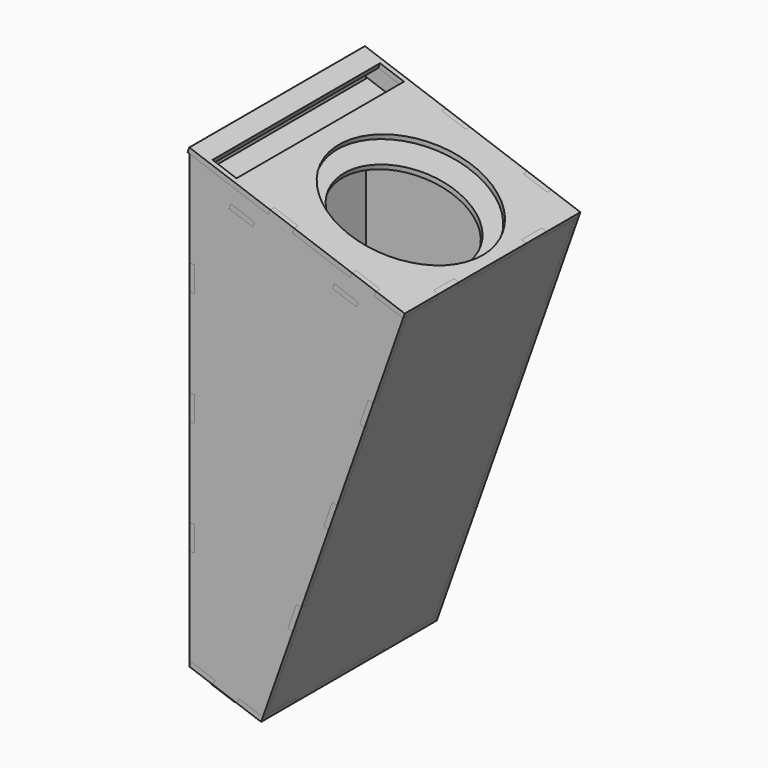
from build123d import *

# Parameters (mm, degrees)
F15_DEPTH = 2
F8_W      = 2
F8_H      = 10
F8_W_2    = 10
F8_H_2    = 2
F16_DEPTH = 2
F11_W     = 2
F11_H     = 10
F11_W_2   = 10
F11_H_2   = 2
F17_DEPTH = 2
F6_R      = 30
F6_W      = 2
F6_H      = 82.4644660941
F6_W_2    = 10
F6_H_2    = 2
F6_W_3    = 15.788135816
F6_W_4    = 24.1412427894
F6_W_5    = 12.0706213947
F6_W_6    = 6
F18_DEPTH = 2
F4_R      = 25
F4_W      = 10
F4_H      = 2
F19_DEPTH = 2
F20_DEPTH = 2
F14_W     = 6
F14_H     = 82.4644660941
F14_H_2   = 20
F21_DEPTH = 2
F22_DEPTH = 2
F23_DEPTH = 2
F24_DEPTH = 2
F25_DEPTH = 2
F26_DEPTH = 2
F27_DEPTH = 2


# Not quite as in the source:
# - a feature names something its author has since deleted; it is built from what else it names


with BuildPart() as f15:
    # F2 (on Front) → F15 (new body)
    with BuildSketch(Plane.XZ):
        Polygon((84.8528137424, 60), (0, 90), (0, -90), (28.2842712475, -100), align=None)
    extrude(amount=F15_DEPTH)


with BuildPart() as f16:
    # F8 (on Right) → F16 (new body)
    with BuildSketch(Plane.YZ):
        Polygon((-2, 40), (-2, 50), (-2, 88), (-16.6161165235, 88), (-26.6161165235, 88), (-59.8483495706, 88), (-69.8483495706, 88), (-84.4644660941, 88), (-84.4644660941, 50), (-84.4644660941, 40), (-84.4644660941, 5), (-84.4644660941, -5), (-84.4644660941, -40), (-84.4644660941, -50), (-84.4644660941, -88), (-69.8483495706, -88), (-59.8483495706, -88), (-26.6161165235, -88), (-16.6161165235, -88), (-2, -88), (-2, -50), (-2, -40), (-2, -5), (-2, 5), align=None)
        with Locations((-1, 45)):
            Rectangle(F8_W, F8_H)
        with Locations((-85.4644660941, 45)):
            Rectangle(F8_W, F8_H)
        with Locations((-85.4644660941, 0)):
            Rectangle(F8_W, F8_H)
        with Locations((-85.4644660941, -45)):
            Rectangle(F8_W, F8_H)
        with Locations((-64.8483495706, -89)):
            Rectangle(F8_W_2, F8_H_2)
        with Locations((-21.6161165235, -89)):
            Rectangle(F8_W_2, F8_H_2)
        with Locations((-1, -45)):
            Rectangle(F8_W, F8_H)
        with Locations((-1, 0)):
            Rectangle(F8_W, F8_H)
    extrude(amount=F16_DEPTH)


with BuildPart() as f17:
    # F11 (on line) → F17 (new body)
    with BuildSketch(Plane(origin=(56.5685424949, 0, -20), x_dir=(0, 1, 0), z_dir=(0.9428090416, 0, -0.3333333333))):
        Polygon((-2, -82.8528137424), (-2, -47.4264068712), (-2, -37.4264068712), (-2, -5), (-2, 5), (-2, 37.4264068712), (-2, 47.4264068712), (-2, 82.8528137424), (-16.6161165235, 82.8528137424), (-26.6161165235, 82.8528137424), (-59.8483495706, 82.8528137424), (-69.8483495706, 82.8528137424), (-84.4644660941, 82.8528137424), (-84.4644660941, 47.4264068712), (-84.4644660941, 37.4264068712), (-84.4644660941, 5), (-84.4644660941, -5), (-84.4644660941, -37.4264068712), (-84.4644660941, -47.4264068712), (-84.4644660941, -82.8528137424), (-69.8483495706, -82.8528137424), (-59.8483495706, -82.8528137424), (-26.6161165235, -82.8528137424), (-16.6161165235, -82.8528137424), align=None)
        with Locations((-85.4644660941, 0)):
            Rectangle(F11_W, F11_H)
        with Locations((-85.4644660941, 42.4264068712)):
            Rectangle(F11_W, F11_H)
        with Locations((-85.4644660941, -42.4264068712)):
            Rectangle(F11_W, F11_H)
        with Locations((-64.8483495706, -83.8528137424)):
            Rectangle(F11_W_2, F11_H_2)
        with Locations((-21.6161165235, -83.8528137424)):
            Rectangle(F11_W_2, F11_H_2)
        with Locations((-1, -42.4264068712)):
            Rectangle(F11_W, F11_H)
        with Locations((-1, 0)):
            Rectangle(F11_W, F11_H)
        with Locations((-1, 42.4264068712)):
            Rectangle(F11_W, F11_H)
        with Locations((-21.6161165235, 83.8528137424)):
            Rectangle(F11_W_2, F11_H_2)
        with Locations((-64.8483495706, 83.8528137424)):
            Rectangle(F11_W_2, F11_H_2)
    extrude(amount=-F17_DEPTH)


with BuildPart() as f18:
    # F6 (on line) → F18 (new body)
    with BuildSketch(Plane(origin=(28.2842712475, 0, 80), x_dir=(0.9428090416, 0, -0.3333333333), z_dir=(0.3333333333, 0, 0.9428090416))):
        Polygon((3.788135816, -2), (-12, -2), (-12, -84.4644660941), (3.788135816, -84.4644660941), (13.788135816, -84.4644660941), (37.9293786053, -84.4644660941), (47.9293786053, -84.4644660941), (60, -84.4644660941), (60, -2), (47.9293786053, -2), (37.9293786053, -2), (13.788135816, -2), align=None)
        with Locations((25.8587572106, -43.232233047)):
            Circle(F6_R, mode=Mode.SUBTRACT)
        with Locations((-29, -43.232233047)):
            Rectangle(F6_W, F6_H)
        Polygon((-28, -84.4644660941), (-30, -84.4644660941), (-30, -86.4644660941), (-22, -86.4644660941), (-22, -84.4644660941), align=None)
        with Locations((-17, -85.4644660941)):
            Rectangle(F6_W_2, F6_H_2)
        with Locations((-4.105932092, -85.4644660941)):
            Rectangle(F6_W_3, F6_H_2)
        with Locations((25.8587572106, -85.4644660941)):
            Rectangle(F6_W_4, F6_H_2)
        with Locations((53.9646893027, -85.4644660941)):
            Rectangle(F6_W_5, F6_H_2)
        with Locations((53.9646893027, -1)):
            Rectangle(F6_W_5, F6_H_2)
        with Locations((25.8587572106, -1)):
            Rectangle(F6_W_4, F6_H_2)
        Polygon((-12, 0), (-12, -2), (3.788135816, -2), (3.788135816, 0), (-10.5049062086, 0), (-11.8180194847, 0), align=None)
        Polygon((-18.1819805153, 0), (-22, 0), (-22, -2), (-12, -2), (-12, 0), (-16.1617604581, 0), align=None)
        Polygon((-22, 0), (-30, 0), (-30, -2), (-28, -2), (-22, -2), align=None)
        with Locations((-25, -43.232233047)):
            Rectangle(F6_W_6, F6_H)
    extrude(amount=-F18_DEPTH)


with BuildPart() as f19:
    # F4 (on line) → F19 (new body)
    with BuildSketch(Plane(origin=(24.9509379141, 0, 70.5719095842), x_dir=(0.9428090416, 0, -0.3333333333), z_dir=(0.3333333333, 0, 0.9428090416))):
        Polygon((0.1516504294, -2), (-9.8483495706, -2), (-24.4644660941, -2), (-24.4644660941, -16.6161165235), (-24.4644660941, -26.6161165235), (-24.4644660941, -59.8483495706), (-24.4644660941, -69.8483495706), (-24.4644660941, -84.4644660941), (-9.8483495706, -84.4644660941), (0.1516504294, -84.4644660941), (33.3838834765, -84.4644660941), (43.3838834765, -84.4644660941), (58, -84.4644660941), (58, -69.8483495706), (58, -59.8483495706), (58, -26.6161165235), (58, -16.6161165235), (58, -2), (43.3838834765, -2), (33.3838834765, -2), align=None)
        with Locations((25.8587572106, -43.232233047)):
            Circle(F4_R, mode=Mode.SUBTRACT)
        with Locations((38.3838834765, -85.4644660941)):
            Rectangle(F4_W, F4_H)
        with Locations((-4.8483495706, -85.4644660941)):
            Rectangle(F4_W, F4_H)
        with Locations((-4.8483495706, -1)):
            Rectangle(F4_W, F4_H)
        with Locations((38.3838834765, -1)):
            Rectangle(F4_W, F4_H)
    extrude(amount=F19_DEPTH)


with BuildPart() as f20:
    # F13 (on line) → F20 (new body)
    with BuildSketch(Plane(origin=(0, -86.4644660941, 0), x_dir=(-1, 0, 0), z_dir=(0, 1, 0))):
        Polygon((0, -90), (0, 90), (-84.8528137424, 60), (-28.2842712475, -100), align=None)
    extrude(amount=F20_DEPTH)


with BuildPart() as f21:
    # F14 (on line) → F21 (new body)
    with BuildSketch(Plane(origin=(-28.2842712475, 0, -80), x_dir=(0.9428090416, 0, -0.3333333333), z_dir=(0.3333333333, 0, 0.9428090416))):
        with Locations((35, -43.232233047)):
            Rectangle(F14_W, F14_H)
        Polygon((38, -84.4644660941), (40, -84.4644660941), (48, -84.4644660941), (48, -2), (40, -2), (38, -2), align=None)
        Polygon((46, -62.4644660941), (46, -82.4644660941), (40, -82.4644660941), (40, -62.4644660941), (40, -24), (40, -4), (46, -4), (46, -24), align=None, mode=Mode.SUBTRACT)
        Polygon((48, -84.4644660941), (50, -84.4644660941), (58, -84.4644660941), (58, -2), (50, -2), (48, -2), align=None)
        Polygon((50, -86.4644660941), (60, -86.4644660941), (60, 0), (50, 0), (50, -2), (58, -2), (58, -84.4644660941), (50, -84.4644660941), align=None)
        Polygon((30, -86.4644660941), (40, -86.4644660941), (40, -84.4644660941), (38, -84.4644660941), (32, -84.4644660941), (32, -2), (38, -2), (40, -2), (40, 0), (30, 0), align=None)
        with Locations((43, -14)):
            Rectangle(F14_W, F14_H_2)
        with Locations((43, -72.4644660941)):
            Rectangle(F14_W, F14_H_2)
    extrude(amount=F21_DEPTH)


with BuildPart() as f22:
    # F14 (on line) → F22 (new body)
    with BuildSketch(Plane(origin=(-28.2842712475, 0, -80), x_dir=(0.9428090416, 0, -0.3333333333), z_dir=(0.3333333333, 0, 0.9428090416))):
        Polygon((38, -84.4644660941), (40, -84.4644660941), (48, -84.4644660941), (48, -2), (40, -2), (38, -2), align=None)
        Polygon((46, -62.4644660941), (46, -82.4644660941), (40, -82.4644660941), (40, -62.4644660941), (40, -24), (40, -4), (46, -4), (46, -24), align=None, mode=Mode.SUBTRACT)
        with Locations((43, -14)):
            Rectangle(F14_W, F14_H_2)
        with Locations((43, -72.4644660941)):
            Rectangle(F14_W, F14_H_2)
    extrude(amount=-F22_DEPTH)


with BuildPart() as f23_tool:
    # F23 (cut): a face of the model
    f23_faces = [f17.part.faces().sort_by_distance(p)[0] for p in [
        (56.5685424949, -43.232233047, -20),
    ]]
    extrude(f23_faces, amount=-F23_DEPTH)


with BuildPart() as f15_1:
    add(f15.part)

    # F23: cut by f23_tool
    add(f23_tool.part, mode=Mode.SUBTRACT)


with BuildPart() as f18_1:
    add(f18.part)

    # F23: cut by f23_tool
    add(f23_tool.part, mode=Mode.SUBTRACT)


with BuildPart() as f20_1:
    add(f20.part)

    # F23: cut by f23_tool
    add(f23_tool.part, mode=Mode.SUBTRACT)


with BuildPart() as f21_1:
    add(f21.part)

    # F23: cut by f23_tool
    add(f23_tool.part, mode=Mode.SUBTRACT)


with BuildPart() as f24_tool:
    # F24 (cut): a face of the model
    f24_faces = [f16.part.faces().sort_by_distance(p)[0] for p in [
        (0, -43.232233047, -0.2426101687),
    ]]
    extrude(f24_faces, amount=-F24_DEPTH)


with BuildPart() as f15_2:
    add(f15_1.part)

    # F24: cut by f24_tool
    add(f24_tool.part, mode=Mode.SUBTRACT)


with BuildPart() as f18_2:
    add(f18_1.part)

    # F24: cut by f24_tool
    add(f24_tool.part, mode=Mode.SUBTRACT)


with BuildPart() as f20_2:
    add(f20_1.part)

    # F24: cut by f24_tool
    add(f24_tool.part, mode=Mode.SUBTRACT)


with BuildPart() as f21_2:
    add(f21_1.part)

    # F24: cut by f24_tool
    add(f24_tool.part, mode=Mode.SUBTRACT)


with BuildPart() as f25_tool:
    # F25 (cut): a face of the model
    f25_faces = [f18_2.part.faces().sort_by_distance(p)[0] for p in [
        (1.1766658696, -43.232233047, 89.5839857922),
    ]]
    extrude(f25_faces, amount=-F25_DEPTH)


with BuildPart() as f15_3:
    add(f15_2.part)

    # F25: cut by f25_tool
    add(f25_tool.part, mode=Mode.SUBTRACT)


with BuildPart() as f16_1:
    add(f16.part)

    # F25: cut by f25_tool
    add(f25_tool.part, mode=Mode.SUBTRACT)


with BuildPart() as f20_3:
    add(f20_2.part)

    # F25: cut by f25_tool
    add(f25_tool.part, mode=Mode.SUBTRACT)


with BuildPart() as f26_tool:
    # F14 (on line) → F26 (new body)
    with BuildSketch(Plane(origin=(-28.2842712475, 0, -80), x_dir=(0.9428090416, 0, -0.3333333333), z_dir=(0.3333333333, 0, 0.9428090416))):
        Polygon((48, -84.4644660941), (50, -84.4644660941), (58, -84.4644660941), (58, -2), (50, -2), (48, -2), align=None)
        Polygon((50, -86.4644660941), (60, -86.4644660941), (60, 0), (50, 0), (50, -2), (58, -2), (58, -84.4644660941), (50, -84.4644660941), align=None)
        Polygon((30, -86.4644660941), (40, -86.4644660941), (40, -84.4644660941), (38, -84.4644660941), (32, -84.4644660941), (32, -2), (38, -2), (40, -2), (40, 0), (30, 0), align=None)
        with Locations((35, -43.232233047)):
            Rectangle(F14_W, F14_H)
    extrude(amount=F26_DEPTH)


with BuildPart() as f15_4:
    add(f15_3.part)

    # F26: cut by f26_tool
    add(f26_tool.part, mode=Mode.SUBTRACT)


with BuildPart() as f20_4:
    add(f20_3.part)

    # F26: cut by f26_tool
    add(f26_tool.part, mode=Mode.SUBTRACT)


with BuildPart() as f27_tool:
    # F27 (cut): a face of the model
    f27_faces = [f19.part.faces().sort_by_distance(p)[0] for p in [
        (9.4423881554, -83.2696233402, 78.1763302781),
    ]]
    extrude(f27_faces, amount=-F27_DEPTH)


with BuildPart() as f15_5:
    add(f15_4.part)

    # F27: cut by f27_tool
    add(f27_tool.part, mode=Mode.SUBTRACT)


with BuildPart() as f16_2:
    add(f16_1.part)

    # F27: cut by f27_tool
    add(f27_tool.part, mode=Mode.SUBTRACT)


with BuildPart() as f20_5:
    add(f20_4.part)

    # F27: cut by f27_tool
    add(f27_tool.part, mode=Mode.SUBTRACT)


solid = Compound([f17.part, f19.part, f22.part, f18_2.part, f21_2.part, f15_5.part, f16_2.part, f20_5.part])
